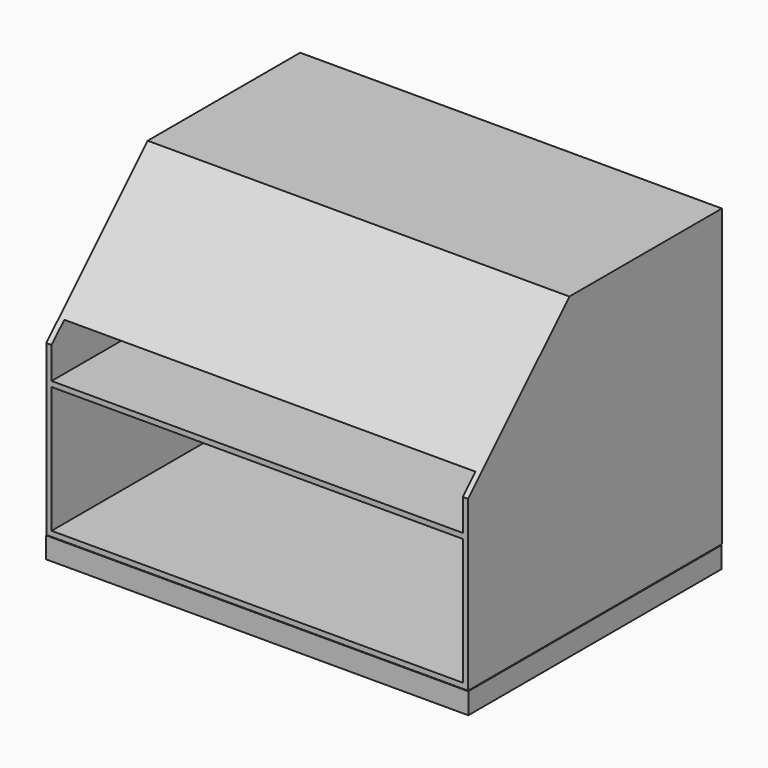
from build123d import *

# Parameters (mm, degrees)
F0_W         = 200
F0_H         = 150
F1_DEPTH     = 10
F2_W         = 199.7782438993
F2_H         = 64.9596797302
F3_DEPTH     = 75
F4_DEPTH     = 75.3
F5_T         = -2.5
F6_DEPTH     = 25
F7_T         = -2.5
F8_W         = 199.7782438993
F8_H         = 150.3
F9_DEPTH     = 50
F10_T1_DEPTH = 508.3802024553
F12_DEPTH    = 9.4


# Not quite as in the source:
# - a fillet or chamfer that OpenCascade refuses, or shapes differently, is made with other operations: its cross-section is extruded or revolved along the edge and cut away or added
# - a shell that OpenCascade refuses in one call is made with other operations: the cavity is built on its own and cut out
# - the program builds the solid bodies; features that only make, move or delete a surface that nothing else refers to are left out


with BuildPart() as f1:
    # F0 (on Top) → F1 (new body)
    with BuildSketch(Plane.XY):
        Rectangle(F0_W, F0_H)
    extrude(amount=F1_DEPTH)


with BuildPart() as f3:
    # F2 (on Front) → F3 (new body)
    with BuildSketch(Plane.XZ):
        with Locations((0, 42.7318564616)):
            Rectangle(F2_W, F2_H)
    extrude(amount=F3_DEPTH)

    # F4 (add): a face of the model
    f4_faces = [f3.faces().sort_by_distance(p)[0] for p in [
        (0, 0, 42.7318564616),
    ]]
    extrude(f4_faces, amount=F4_DEPTH)

    # F5
    f5_openings = [f3.faces().sort_by_distance(p)[0] for p in [
        (0, -75, 42.731856),
    ]]
    offset(amount=F5_T, openings=f5_openings)

    # F6 (add): a face of the model
    f6_faces = [f3.faces().sort_by_distance(p)[0] for p in [
        (0, 0.15, 75.2116963267),
    ]]
    extrude(f6_faces, amount=F6_DEPTH)

    # F7: a shell. OpenCascade refuses it in one call, so the cavity is built on its own and cut out:
    # the body offset inwards by the wall thickness, plus a prism from it out through each open face.
    f7_core = offset(f3.part, amount=F7_T, kind=Kind.INTERSECTION, mode=Mode.PRIVATE)
    f7_exits = [f7_core.faces().sort_by_distance(p)[0] for p in [
        (0, -72.5, 86.461696),
    ]]
    add(f7_core, mode=Mode.SUBTRACT)
    extrude(f7_exits, amount=-F7_T, mode=Mode.SUBTRACT)

    # F8 (on face) → F9 (join)
    with BuildSketch(Plane.XY.offset(100.2116963267)):
        with Locations((0, 0.15)):
            Rectangle(F8_W, F8_H)
    extrude(amount=F9_DEPTH)

    # F10: chamfer of 60 on 1 edges, made by hand

    # F10_s2 → F10_t1 (cut)
    with BuildSketch(Plane.YZ.offset(-254.1901012276)):
        Polygon((-15, 150.2116963267), (-75, 90.2116963267), (-75, 150.2116963267), align=None)
    extrude(amount=F10_T1_DEPTH, mode=Mode.SUBTRACT)

    # F11 (on face) → F12 (join)
    with BuildSketch(Plane(origin=(0, -82.6058481634, 82.6058481634), x_dir=(1, 0, 0), z_dir=(0, -0.7071067812, 0.7071067812))):
        Polygon((76.5384733677, 70.738479495), (-67.3584118485, 70.738479495), (76.5384733677, 43.4501171112), align=None)
    extrude(amount=-F12_DEPTH)


solid = Compound([f1.part, f3.part])
